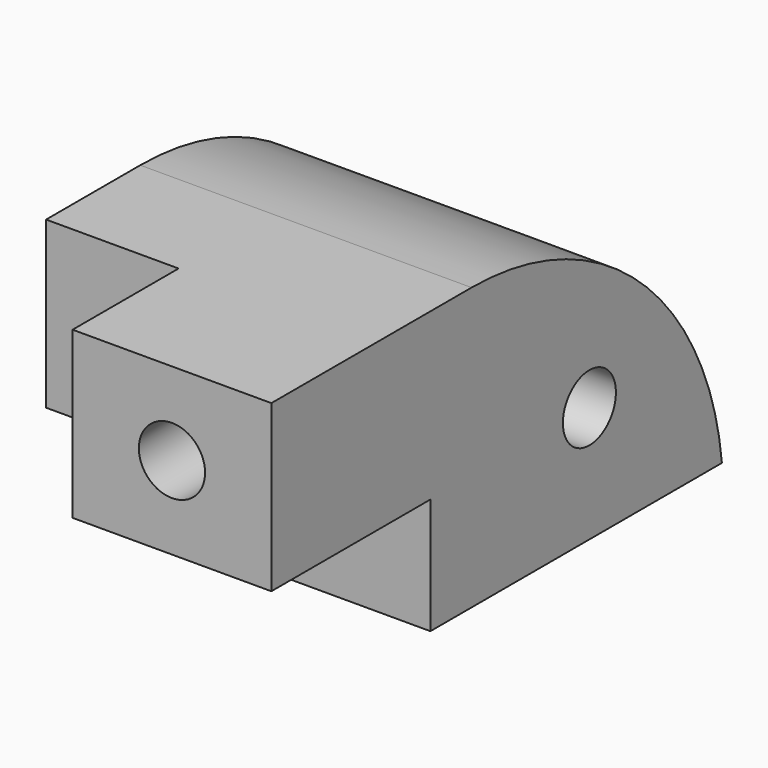
from build123d import *

# Parameters (mm, degrees)
F0_W        = 127
F0_H        = 139.7
F1_DEPTH    = 107.95
F2_T1_DEPTH = 726.8985851792
F3_W        = 127
F3_H        = 63.5
F4_DEPTH    = 25.4
F5_W        = 76.2
F5_H        = 63.5
F6_DEPTH    = 50.8
F8_D        = 25.4
F10_D       = 25.4


# Not quite as in the source:
# - a fillet or chamfer that OpenCascade refuses, or shapes differently, is made with other operations: its cross-section is extruded or revolved along the edge and cut away or added


with BuildPart() as f1:
    # F0 (on Top) → F1 (new body)
    with BuildSketch(Plane.XY):
        with Locations((-63.5, 4.4167287707)):
            Rectangle(F0_W, F0_H)
    extrude(amount=F1_DEPTH)

    # F2: fillet of radius 120.65 on 1 edges, made by hand

    # F2_s2 → F2_t1 (cut)
    with BuildSketch(Plane.YZ.offset(-426.9492925896)):
        with BuildLine():
            ThreePointArc((74.2667287707, 0), (34.9844946572, 76.9902377631), (-45.7129882651, 107.95))
            Line((-45.7129882651, 107.95), (74.2667287707, 107.95))
            Line((74.2667287707, 107.95), (74.2667287707, 0))
        make_face()
    extrude(amount=F2_T1_DEPTH, mode=Mode.SUBTRACT)

    # F3 (on face) → F4 (join)
    with BuildSketch(Plane.XZ.offset(65.4332712293)):
        with Locations((-63.5, 76.2)):
            Rectangle(F3_W, F3_H)
    extrude(amount=F4_DEPTH)

    # F5 (on face) → F6 (join)
    with BuildSketch(Plane.XZ.offset(90.8332712293)):
        with Locations((-38.1, 76.2)):
            Rectangle(F5_W, F5_H)
    extrude(amount=F6_DEPTH)

    # F8 (through all)
    with Locations(Plane.XZ.offset(141.6332712293)):
        with Locations((-38.1, 76.2)):
            Hole(F8_D / 2)

    # F10 (through all)
    with Locations(Plane.YZ):
        with Locations((10.7667287707, 44.45)):
            Hole(F10_D / 2)


solid = f1.part
